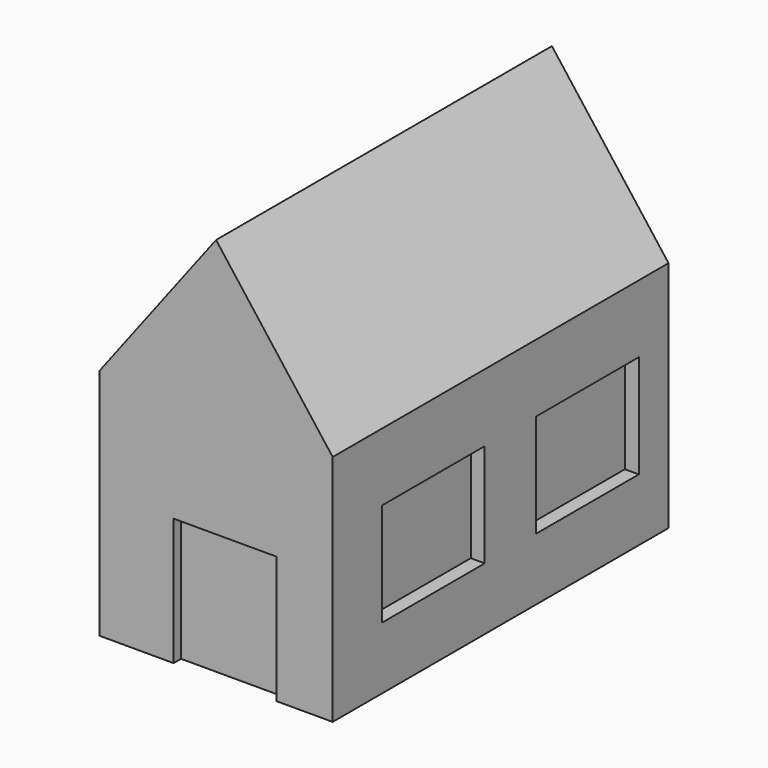
from build123d import *

# Parameters (mm, degrees)
F0_W      = 127
F0_H      = 127
F1_DEPTH  = 127
F2_DEPTH  = 25.4
F3_DEPTH  = 76.2
F5_DEPTH  = 228.6
F6_W      = 55.9784695506
F6_H      = 69.2825764418
F7_DEPTH  = 5.08
F8_W      = 69.8941033334
F8_H      = 56.1961345005
F9_DEPTH  = 7.62
F11_W     = 69.8941033334
F11_H     = 56.1961345005
F10_W     = 69.8941033334
F10_H     = 56.1961345005
F12_DEPTH = 7.62
F13_T     = -5.08


# Not quite as in the source:
# - a shell that OpenCascade refuses in one call is made with other operations: the cavity is built on its own and cut out


with BuildPart() as f1:
    # F0 (on Top) → F1 (new body)
    with BuildSketch(Plane.XY):
        with Locations((63.5, -63.5)):
            Rectangle(F0_W, F0_H)
    extrude(amount=F1_DEPTH)

    # F2 (add): a face of the model
    f2_faces = [f1.faces().sort_by_distance(p)[0] for p in [
        (63.5, -127, 63.5),
    ]]
    extrude(f2_faces, amount=F2_DEPTH)

    # F3 (add): a face of the model
    f3_faces = [f1.faces().sort_by_distance(p)[0] for p in [
        (63.5, -152.4, 63.5),
    ]]
    extrude(f3_faces, amount=F3_DEPTH)

    # F4 (on face) → F5 (join)
    with BuildSketch(Plane.XZ.offset(228.6)):
        Polygon((63.5, 210.3958427906), (63.5, 127), (127, 127), align=None)
        Polygon((63.5, 210.3958427906), (0, 127), (63.5, 127), align=None)
    extrude(amount=-F5_DEPTH)

    # F6 (on face) → F7 (cut)
    with BuildSketch(Plane.XZ.offset(228.6)):
        with Locations((68.3894939721, 34.6412882209)):
            Rectangle(F6_W, F6_H)
    extrude(amount=-F7_DEPTH, mode=Mode.SUBTRACT)

    # F8 (on face) → F9 (cut)
    with BuildSketch(Plane(origin=(0, 0, 0), x_dir=(0, -1, 0), z_dir=(-1, 0, 0))):
        with Locations((55.1468739286, 62.0407964849)):
            Rectangle(F8_W, F8_H)
        with Locations((160.0488739286, 62.0407964849)):
            Rectangle(F8_W, F8_H)
    extrude(amount=-F9_DEPTH, mode=Mode.SUBTRACT)

    # F11 (on face) + F10 (on face) → F12 (cut)
    with BuildSketch(Plane.YZ.offset(127)):
        with Locations((-160.0488739286, 62.0407964849)):
            Rectangle(F11_W, F11_H)
    with BuildSketch(Plane.YZ.offset(127)):
        with Locations((-55.1468739286, 62.0407964849)):
            Rectangle(F10_W, F10_H)
    extrude(amount=-F12_DEPTH, mode=Mode.SUBTRACT)

    # F13: a shell. OpenCascade refuses it in one call, so the cavity is built on its own and cut out:
    # the body offset inwards by the wall thickness, plus a prism from it out through each open face.
    f13_core = offset(f1.part, amount=F13_T, kind=Kind.INTERSECTION, mode=Mode.PRIVATE)
    f13_exits = [f13_core.faces().sort_by_distance(p)[0] for p in [
        (63.434775, -112.87691, 5.08),
    ]]
    add(f13_core, mode=Mode.SUBTRACT)
    extrude(f13_exits, amount=-F13_T, mode=Mode.SUBTRACT)


solid = f1.part
